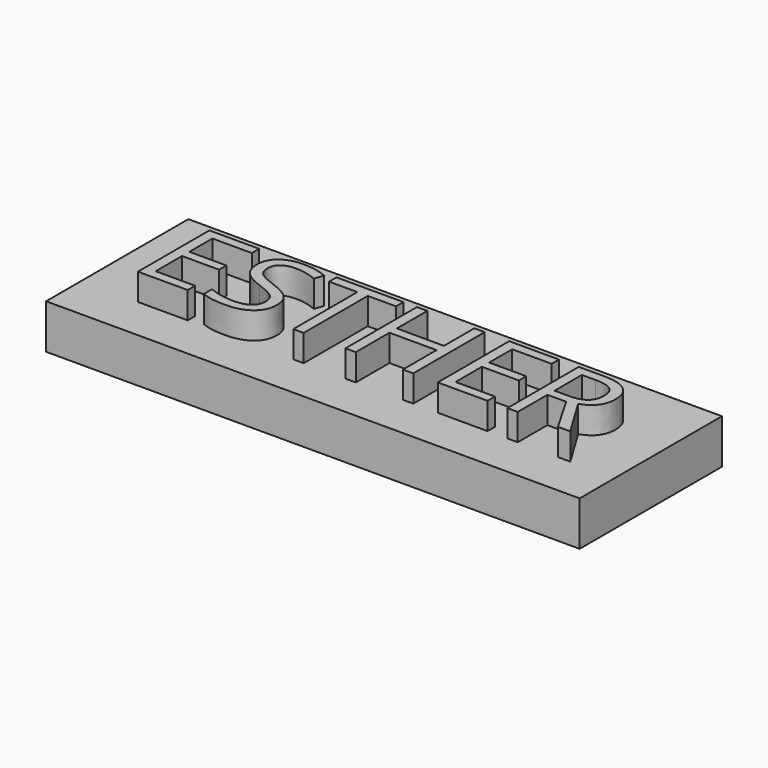
from build123d import *

# Parameters (mm, degrees)
F0_W         = 60
F0_H         = 20
F1_DEPTH     = 5
F2_TEXT_SIZE = 14.0715008135
F3_DEPTH     = 3


# Not quite as in the source:
# - Text() gives the source's letters only with a copy of the font that has no kerning and outlines rounded to 1/6400 em; it was checked with that copy


with BuildPart() as f1:
    # F0 (on Top) → F1 (new body)
    with BuildSketch(Plane.XY):
        Rectangle(F0_W, F0_H)
    extrude(amount=F1_DEPTH)

    # F2 (on face) → F3 (join)
    with BuildSketch(Plane.XY.offset(5)):
        with Locations((-25, -5.0659805857)):
            Text('ESTHER', F2_TEXT_SIZE, font='Open Sans', text_align=(TextAlign.LEFT, TextAlign.BOTTOM))
    extrude(amount=F3_DEPTH)


solid = f1.part
